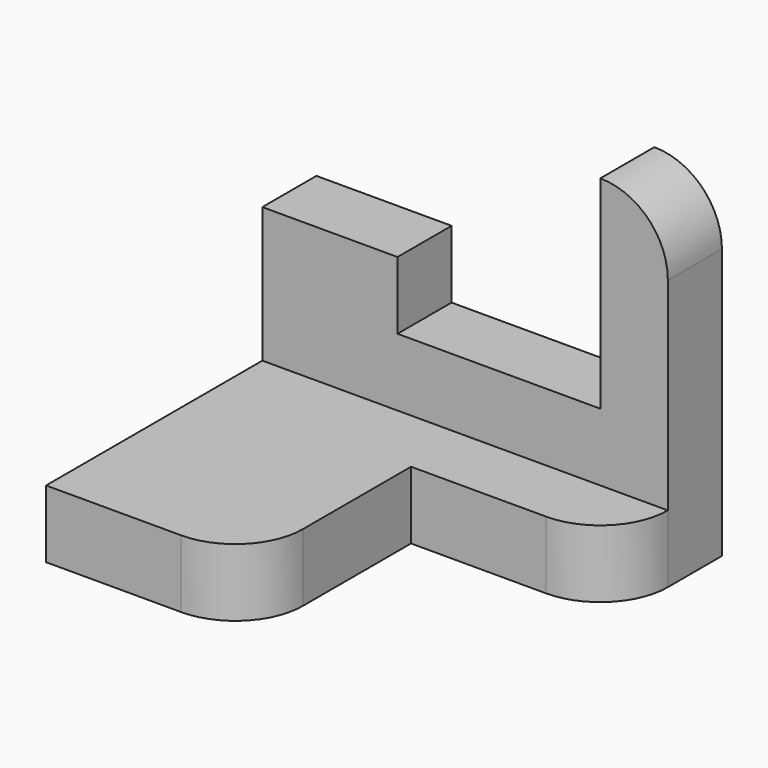
from build123d import *

# Parameters (mm, degrees)
F1_DEPTH = 10
F3_DEPTH = 10


# Not quite as in the source:
# - a feature names something its author has since deleted; it is built from what else it names


with BuildPart() as f1:
    # F0 (on Top) → F1 (new body)
    with BuildSketch(Plane.XY):
        with BuildLine():
            Line((60, 0), (20, 0))
            Line((20, 0), (0, 0))
            Line((0, 0), (0, -50))
            Line((0, -50), (20, -50))
            ThreePointArc((20, -50), (27.0710678119, -47.0710678119), (30, -40))
            Line((30, -40), (30, -20))
            Line((30, -20), (50, -20))
            ThreePointArc((50, -20), (57.0710678119, -17.0710678119), (60, -10))
            Line((60, -10), (60, 0))
        make_face()
    extrude(amount=F1_DEPTH)

    # F2 (on Front) → F3 (join)
    with BuildSketch(Plane.XZ):
        with BuildLine():
            Line((0, 30), (0, 10))
            Line((0, 10), (60, 10))
            Line((60, 10), (60, 40))
            ThreePointArc((60, 40), (57.0710678119, 47.0710678119), (50, 50))
            Line((50, 50), (50, 20))
            Line((50, 20), (20, 20))
            Line((20, 20), (20, 30))
            Line((20, 30), (0, 30))
        make_face()
    extrude(amount=F3_DEPTH)


solid = f1.part
